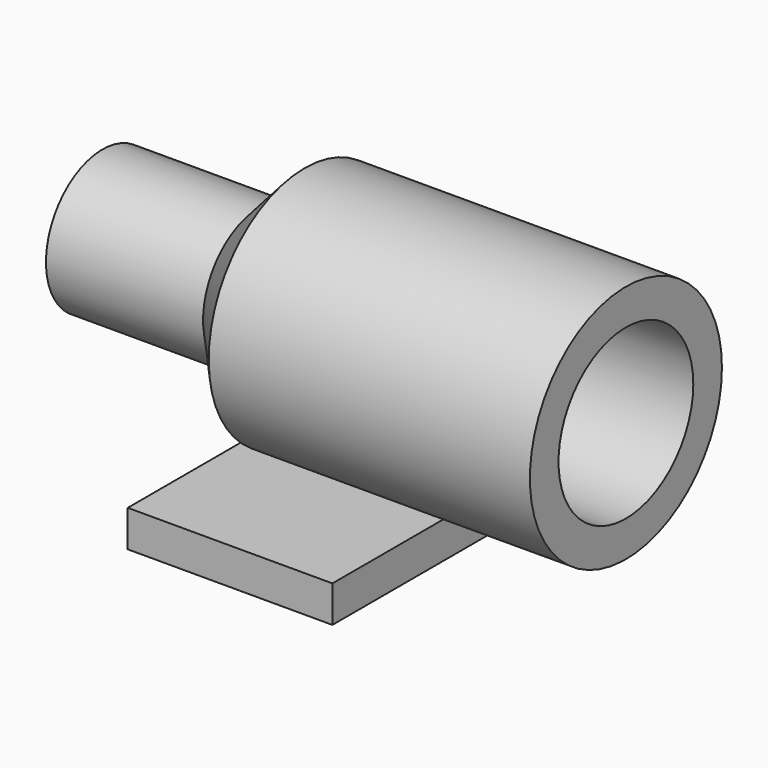
from build123d import *

# Parameters (mm, degrees)
F2_W     = 49.1305962205
F2_H     = 4.4664181769
F3_DEPTH = 12.5


# Not quite as in the source:
# - a feature names something its author has since deleted; it is built from what else it names


with BuildPart() as f1:
    # F0 (on Top) → F1 (revolve)
    with BuildSketch(Plane.XY):
        Polygon((-35.6138087809, 8.6301378906), (-35.6138087809, 3.1164383981), (-16.4602123841, 3.1164383981), (-13.8548975913, 5.887503858), (-10.9075363725, 3.1164383981), (-4.8190304078, 3.1164383981), (-4.8190304078, 10.2874673903), (28.3264927566, 10.2874673903), (28.3264927566, 14.6608594805), (-10.9075363725, 14.6608594805), (-16.4212342352, 8.6301378906), align=None)
    revolve(axis=Axis((-1.5279836953, 0, 0), (1, 0, 0)))

    # F2 (on Right) → F3 (join, symmetric)
    with BuildSketch(Plane.YZ):
        with Locations((-0.4701502621, -14.4570898265)):
            Rectangle(F2_W, F2_H)
    extrude(amount=F3_DEPTH, both=True)


solid = f1.part
